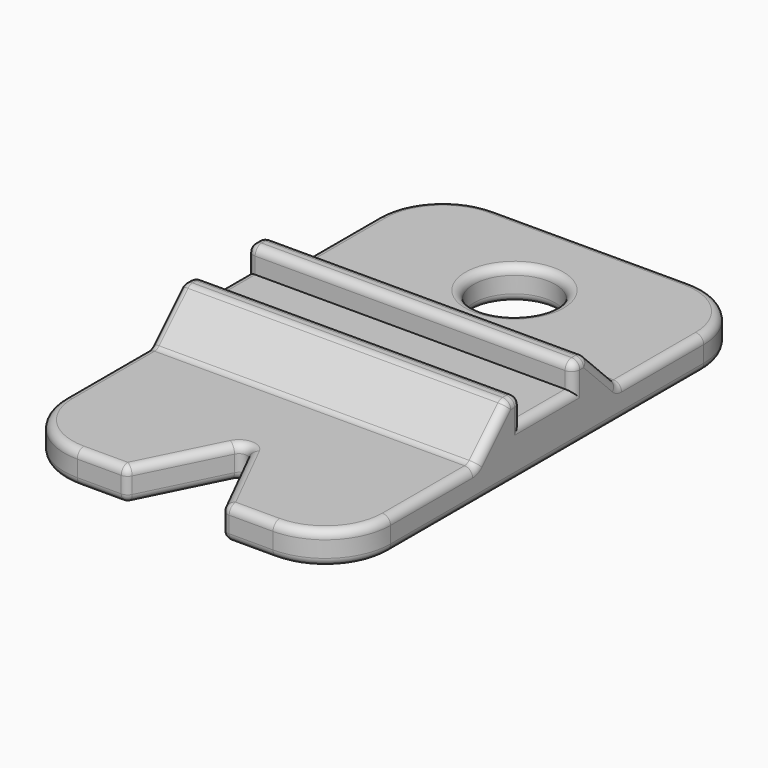
from build123d import *

# Parameters (mm, degrees)
F0_W          = 127
F0_H          = 203.2
F1_DEPTH      = 12.7
F2_R          = 15.875
F3_DEPTH      = 25.4
F5_DEPTH      = 25.4
F7_DEPTH      = 63.5
F7_DEPTH_BACK = 63.5
F8_R          = 25.4
F9_R          = 3.175


# Not quite as in the source:
# - a feature of the source that left no trace in its solid (it failed there, or was rolled back) is left out
# - a feature names something its author has since deleted; it is built from what else it names


with BuildPart() as f1:
    # F0 (on Top) → F1 (new body)
    with BuildSketch(Plane.XY):
        with Locations((0, -38.1)):
            Rectangle(F0_W, F0_H)
    extrude(amount=F1_DEPTH)

    # F2 (on Top) → F3 (cut)
    with BuildSketch(Plane.XY):
        with Locations((0, 25.4)):
            Circle(F2_R)
    extrude(amount=F3_DEPTH, mode=Mode.SUBTRACT)

    # F4 (on Top) → F5 (cut)
    with BuildSketch(Plane.XY):
        Polygon((38.1, -177.8), (0, -101.6), (-38.1, -177.8), align=None)
    extrude(amount=F5_DEPTH, mode=Mode.SUBTRACT)

    # F6 (on Right) → F7 (join, two sides)
    with BuildSketch(Plane.YZ) as f7_sk:
        Polygon((9.525, 0), (-19.05, 28.575), (-25.4, 28.575), (-25.4, 19.05), (-50.8, 19.05), (-50.8, 28.575), (-57.15, 28.575), (-85.725, 0), align=None)
    extrude(amount=F7_DEPTH)
    extrude(f7_sk.sketch, amount=-F7_DEPTH_BACK)

    # F8
    f8_edges = [f1.edges().sort_by_distance(p)[0] for p in [
        (63.5, -139.7, 6.35),
        (-63.5, -139.7, 6.35),
        (-63.5, 63.5, 6.35),
        (63.5, 63.5, 6.35),
    ]]
    fillet(f8_edges, radius=F8_R)

    # F9
    f9_edges = [f1.edges().sort_by_distance(p)[0] for p in [
        (-19.05, -139.7, 6.35),
        (19.05, -139.7, 6.35),
        (0, -101.6, 6.35),
        (0, -50.8, 28.575),
        (0, -25.4, 28.575),
        (0, 63.5, 0),
        (0, 63.5, 12.7),
        (-63.5, -38.1, 0),
        (-56.060512, 56.060512, 0),
        (-56.060512, -132.260512, 0),
        (-28.575, -139.7, 0),
        (56.060512, 56.060512, 0),
        (-9.525, -120.65, 0),
        (63.5, -38.1, 0),
        (9.525, -120.65, 0),
        (56.060512, -132.260512, 0),
        (28.575, -139.7, 0),
        (-15.875, 25.4, 0),
        (56.060512, 56.060512, 12.7),
        (-56.060512, 56.060512, 12.7),
        (-63.5, 17.4625, 12.7),
        (0, -3.175, 12.7),
        (63.5, 17.4625, 12.7),
        (-15.875, 25.4, 12.7),
        (-63.5, -93.6625, 12.7),
        (-63.5, -11.1125, 20.6375),
        (-63.5, -65.0875, 20.6375),
        (-63.5, -22.225, 28.575),
        (-63.5, -53.975, 28.575),
        (-63.5, -25.4, 23.8125),
        (-63.5, -50.8, 23.8125),
        (-63.5, -38.1, 19.05),
        (-56.060512, -132.260512, 12.7),
        (-28.575, -139.7, 12.7),
        (-9.525, -120.65, 12.7),
        (63.5, -93.6625, 12.7),
        (63.5, -65.0875, 20.6375),
        (63.5, -11.1125, 20.6375),
        (63.5, -53.975, 28.575),
        (63.5, -22.225, 28.575),
        (63.5, -50.8, 23.8125),
        (63.5, -25.4, 23.8125),
        (63.5, -38.1, 19.05),
        (9.525, -120.65, 12.7),
        (56.060512, -132.260512, 12.7),
        (28.575, -139.7, 12.7),
        (0, -19.05, 28.575),
        (0, -73.025, 12.7),
        (0, -57.15, 28.575),
    ]]
    fillet(f9_edges, radius=F9_R)


solid = f1.part
